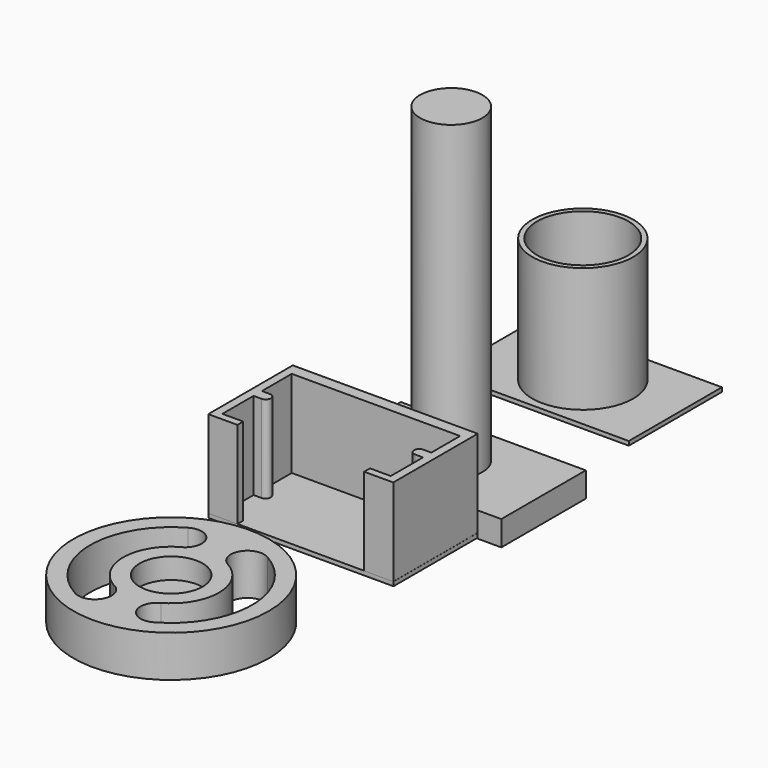
from build123d import *

# Parameters (mm, degrees)
F2_DEPTH  = 21
F0_W      = 44.5381999016
F0_H      = 25.3221206367
F3_DEPTH  = 1
F1_W      = 44.5
F1_H      = 25.4
F4_DEPTH  = 6
F5_R      = 7.5
F6_DEPTH  = 75
F7_R      = 23.5
F8_DEPTH  = 10
F10_D     = 8
F12_DEPTH = 25
F13_W     = 44.538
F13_H     = 28
F13_R     = 11
F14_DEPTH = 1
F15_R     = 12.1568017558
F15_R_2   = 11
F16_DEPTH = 30
F17_R     = 7.575
F18_DEPTH = 5


with BuildPart() as f2:
    # F1 (on Top) → F2 (new body)
    with BuildSketch(Plane.XY):
        with BuildLine():
            Line((-19.25, 9.9), (20.25, 9.9))
            Line((20.25, 9.9), (20.25, 1.25))
            Line((20.25, 1.25), (18.35, 1.25))
            ThreePointArc((18.35, 1.25), (17.1, 0), (18.35, -1.25))
            Line((18.35, -1.25), (20.25, -1.25))
            Line((20.25, -1.25), (20.25, -9.7038764507))
            Line((20.25, -9.7038764507), (20.25, -10.95))
            Line((20.25, -10.95), (15.25, -10.95))
            Line((15.25, -10.95), (15.25, -12.7))
            Line((15.25, -12.7), (22.25, -12.7))
            Line((22.25, -12.7), (22.25, 12.7))
            Line((22.25, 12.7), (-22.25, 12.7))
            Line((-22.25, 12.7), (-22.25, -12.7))
            Line((-22.25, -12.7), (-15.25, -12.7))
            Line((-15.25, -12.7), (-15.25, -10.95))
            Line((-15.25, -10.95), (-20.25, -10.95))
            Line((-20.25, -10.95), (-20.25, -9.7))
            Line((-20.25, -9.7), (-20.25, -1.5828977921))
            Line((-20.25, -1.5828977921), (-18.35, -1.5828977921))
            ThreePointArc((-18.35, -1.5828977921), (-17.0996297668, -0.3325275589), (-18.35, 0.9178426743))
            Line((-18.35, 0.9178426743), (-20.25, 0.9178426743))
            Line((-20.25, 0.9178426743), (-20.25, 9.9))
            Line((-20.25, 9.9), (-19.25, 9.9))
        make_face()
    extrude(amount=F2_DEPTH)

    # F0 (on Top) → F3 (join)
    with BuildSketch(Plane.XY):
        Rectangle(F0_W, F0_H)
    extrude(amount=-F3_DEPTH)


with BuildPart() as f4:
    # F1 (on Top) → F4 (new body)
    with BuildSketch(Plane.XY):
        with Locations((-0.040480867, 32.5438007712)):
            Rectangle(F1_W, F1_H)
    extrude(amount=-F4_DEPTH)

    # F5 (on face) → F6 (join)
    with BuildSketch(Plane.XY):
        with Locations((0, 32.5438007712)):
            Circle(F5_R)
    extrude(amount=F6_DEPTH)


with BuildPart() as f8:
    # F7 (on Top) → F8 (new body)
    with BuildSketch(Plane.XY):
        with Locations((0, -51.663291269)):
            Circle(F7_R)
    extrude(amount=F8_DEPTH)

    # F10 (through all)
    with Locations(Plane(origin=(0, 0, 0), x_dir=(1, 0, 0), z_dir=(0, 0, -1))):
        with Locations((-7.5, 38.0986313028), (7.5, 38.0986313028), (-7.5, 65.2279512353), (7.5, 65.2279512353)):
            Hole(F10_D / 2)

    # F11 (on face) → F12 (cut)
    with BuildSketch(Plane.XY.offset(10)):
        with BuildLine():
            ThreePointArc((11.5, -65.2279512353), (11.007417817, -67.1509749628), (9.6509898716, -68.6003750776))
            ThreePointArc((9.6509898716, -68.6003750776), (19.4937531902, -51.663291269), (9.6509898716, -34.7262074605))
            ThreePointArc((9.6509898716, -34.7262074605), (4.0651326687, -36.0488297473), (5.5531980506, -41.5929069315))
            ThreePointArc((5.5531980506, -41.5929069315), (11.500020945, -51.6503468012), (5.5758544768, -61.7211487022))
            ThreePointArc((5.5758544768, -61.7211487022), (9.5375742818, -61.7858165711), (11.5, -65.2279512353))
        make_face()
        with BuildLine():
            ThreePointArc((-9.5496674592, -68.6628985867), (-11.0797578572, -63.4432009211), (-5.9903344615, -61.5237765685))
            ThreePointArc((-5.9903344615, -61.5237765685), (-11.5374727433, -51.663291269), (-5.9903344615, -41.8028059695))
            ThreePointArc((-5.9903344615, -41.8028059695), (-11.0797578572, -39.8833816169), (-9.5496674592, -34.6636839514))
            ThreePointArc((-9.5496674592, -34.6636839514), (-19.4982767837, -51.663291269), (-9.5496674592, -68.6628985867))
        make_face()
    extrude(amount=-F12_DEPTH, mode=Mode.SUBTRACT)

    # F17 (on face) → F18 (cut)
    with BuildSketch(Plane.XY.offset(10)):
        with Locations((0, -51.663291269)):
            Circle(F17_R)
    extrude(amount=-F18_DEPTH, mode=Mode.SUBTRACT)


with BuildPart() as f14:
    # F13 (on Top) → F14 (new body)
    with BuildSketch(Plane.XY):
        with Locations((0, 72.1066973255)):
            Rectangle(F13_W, F13_H)
        with Locations((0, 72.1066973255)):
            Circle(F13_R, mode=Mode.SUBTRACT)
    extrude(amount=F14_DEPTH)

    # F15 (on face) → F16 (join)
    with BuildSketch(Plane.XY.offset(1)):
        with Locations((0, 72.1066973255)):
            Circle(F15_R)
        with Locations((0, 72.1066973255)):
            Circle(F15_R_2, mode=Mode.SUBTRACT)
    extrude(amount=F16_DEPTH)


solid = Compound([f2.part, f4.part, f8.part, f14.part])
